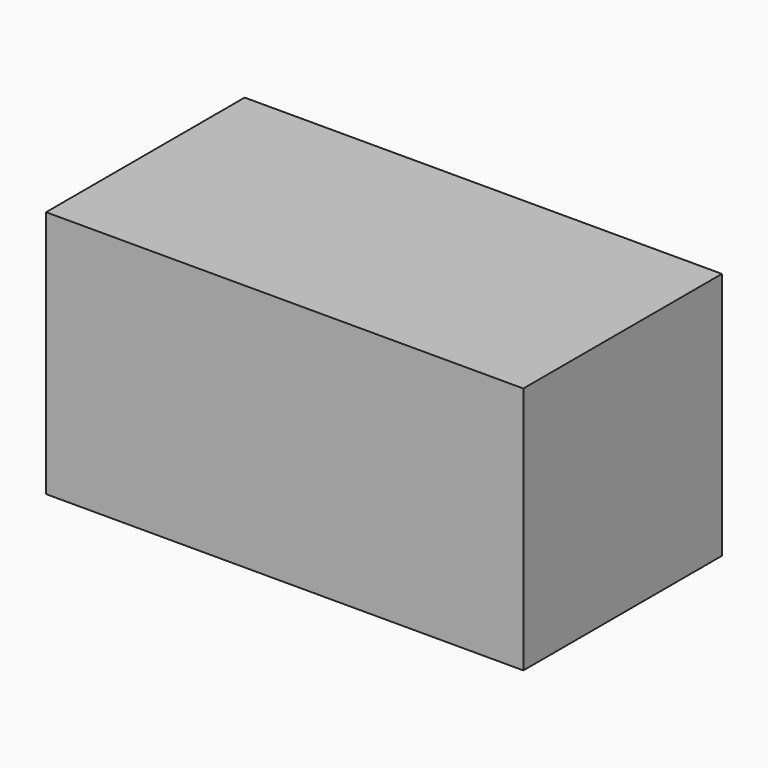
from build123d import *

# Parameters (mm, degrees)
F1_E0_W  = 4.8840213567
F1_E0_H  = 2.54
F2_DEPTH = 2.54


with BuildPart() as f2:
    # F1_E0 (on explicit) → F2 (new body)
    with BuildSketch(Plane(origin=(0, 1.27, 0), x_dir=(1, 0, 0), z_dir=(0, 0, -1))):
        with Locations((2.4420106784, 1.27)):
            Rectangle(F1_E0_W, F1_E0_H)
    extrude(amount=F2_DEPTH)


solid = f2.part
